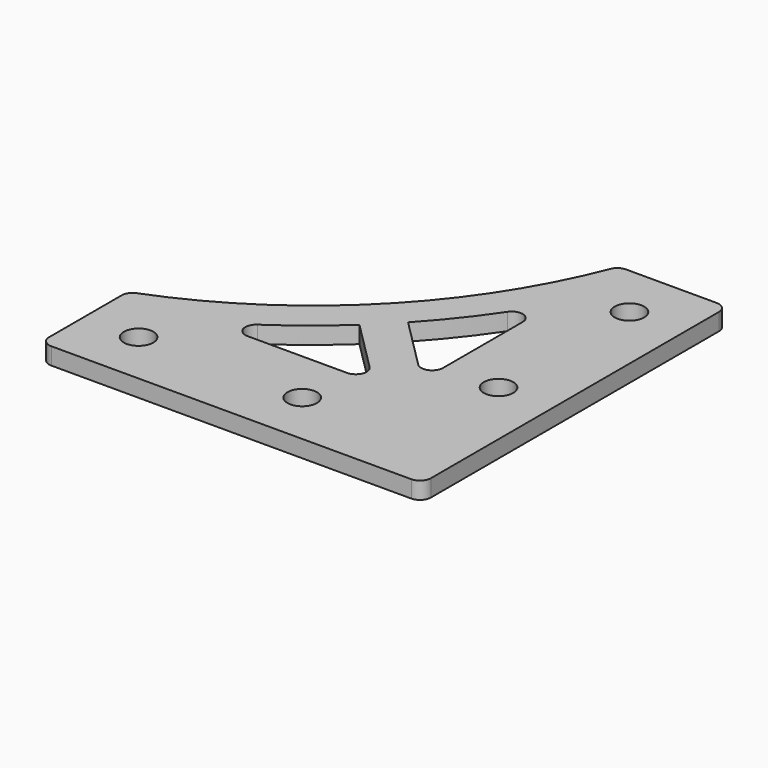
from build123d import *

# Parameters (mm, degrees)
F1_DEPTH = 3.125
F2_W     = 6
F2_H     = 50
F2_W_2   = 50
F2_H_2   = 6
F3_DEPTH = 2
F4_R     = 2.7
F5_DEPTH = 25
F6_R     = 2
F8_DEPTH = 25
F9_R     = 2


# Not quite as in the source:
# - a feature names something its author has since deleted; it is built from what else it names


with BuildPart() as f1:
    # F0 (on Top) → F1 (new body)
    with BuildSketch(Plane.XY):
        with BuildLine():
            Line((35, 35), (15, 35))
            ThreePointArc((15, 35), (-4.5539513718, 4.5539513718), (-35, -15))
            Line((-35, -15), (-35, -35))
            Line((-35, -35), (35, -35))
            Line((35, -35), (35, 35))
        make_face()
    extrude(amount=F1_DEPTH)

    # F2 (on face) → F3 (join)
    with BuildSketch(Plane(origin=(0, 0, 0), x_dir=(1, 0, 0), z_dir=(0, 0, -1))):
        with Locations((25, -10)):
            Rectangle(F2_W, F2_H)
        with Locations((-10, 25)):
            Rectangle(F2_W_2, F2_H_2)
    extrude(amount=F3_DEPTH)

    # F4 (on face) → F5 (cut)
    with BuildSketch(Plane(origin=(0, 0, -2), x_dir=(1, 0, 0), z_dir=(0, 0, -1))):
        with Locations((25, -25)):
            Circle(F4_R)
        with Locations((25, 5)):
            Circle(F4_R)
        with Locations((5, 25)):
            Circle(F4_R)
        with Locations((-25, 25)):
            Circle(F4_R)
    extrude(amount=-F5_DEPTH, mode=Mode.SUBTRACT)

    # F6
    f6_edges = [f1.edges().sort_by_distance(p)[0] for p in [
        (35, 35, 1.5625),
        (15, 35, 1.5625),
        (-35, -15, 1.5625),
        (-35, -35, 1.5625),
        (35, -35, 1.5625),
    ]]
    fillet(f6_edges, radius=F6_R)

    # F7 (on Top) → F8 (cut)
    with BuildSketch(Plane.XY):
        with BuildLine():
            Line((15, -10.0502525317), (15, 20))
            ThreePointArc((15, 20), (9.1151461726, 10.9887424757), (2.2488038315, 2.7009436368))
            Line((2.2488038315, 2.7009436368), (15, -10.0502525317))
        make_face()
        with BuildLine():
            ThreePointArc((-2.7009436368, -2.2488038315), (-10.9887424757, -9.1151461726), (-20, -15))
            Line((-20, -15), (10.0502525317, -15))
            Line((10.0502525317, -15), (-2.7009436368, -2.2488038315))
        make_face()
    extrude(amount=F8_DEPTH, mode=Mode.SUBTRACT)

    # F9
    f9_edges = [f1.edges().sort_by_distance(p)[0] for p in [
        (15, 20, 1.5625),
        (-20, -15, 1.5625),
        (10.050253, -15, 1.5625),
        (15, -10.050253, 1.5625),
    ]]
    fillet(f9_edges, radius=F9_R)


solid = f1.part
